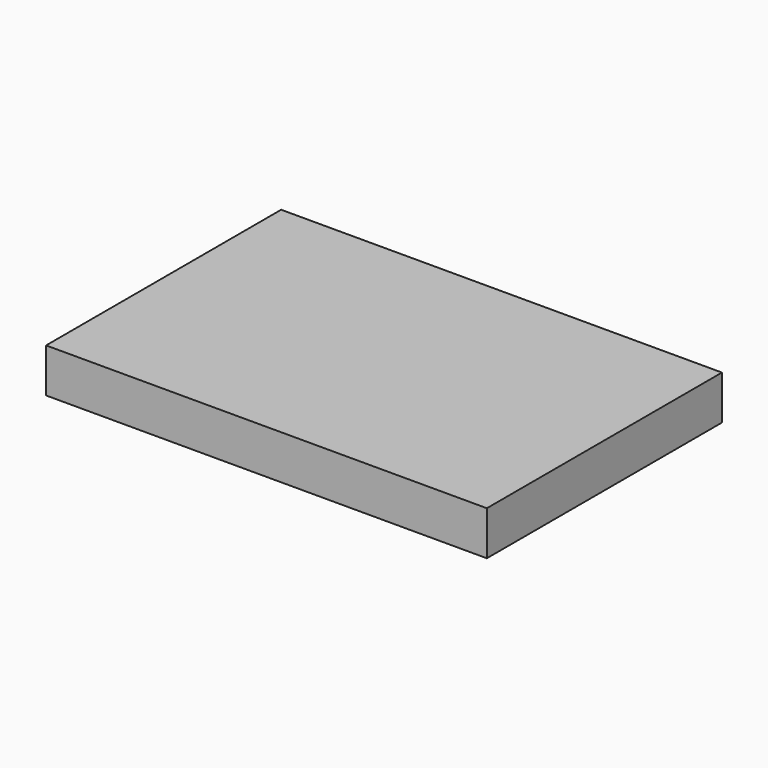
from build123d import *

# Parameters (mm, degrees)
F0_W     = 150
F0_H     = 100
F1_DEPTH = 15


# Not quite as in the source:
# - the program builds the solid bodies; features that only make, move or delete a surface that nothing else refers to are left out


with BuildPart() as f1:
    # F0 (on Top) → F1 (new body)
    with BuildSketch(Plane.XY):
        Rectangle(F0_W, F0_H)
    extrude(amount=F1_DEPTH)


solid = f1.part
